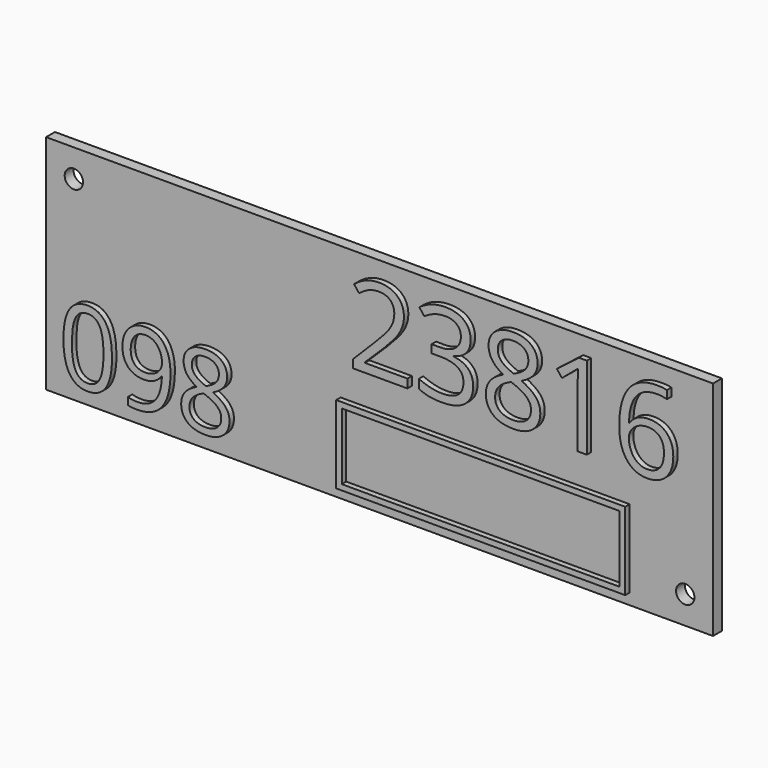
from build123d import *

# Parameters (mm, degrees)
F0_W         = 120
F0_H         = 40
F1_DEPTH     = 2
F3_D         = 3.3
F4_TEXT_SIZE = 20.871833895
F5_DEPTH     = 1
F6_TEXT_SIZE = 18.5155049272
F7_DEPTH     = 1
F8_W         = 52
F8_H         = 14
F8_W_2       = 49.99999962
F8_H_2       = 11.99999962
F9_DEPTH     = 1


# Not quite as in the source:
# - Text() gives the source's letters only with a copy of the font that has no kerning and outlines rounded to 1/6400 em; it was checked with that copy


with BuildPart() as f1:
    # F0 (on Front) → F1 (new body)
    with BuildSketch(Plane.XZ):
        Rectangle(F0_W, F0_H)
    extrude(amount=F1_DEPTH)

    # F3 (through all)
    with Locations(Plane.XZ.offset(2)):
        with Locations((-55, 15), (55, -15)):
            Hole(F3_D / 2)

    # F4 (on face) → F5 (join)
    with BuildSketch(Plane.XZ.offset(2)):
        with Locations((-5, 2)):
            Text('23816', F4_TEXT_SIZE, font='Open Sans', text_align=(TextAlign.LEFT, TextAlign.BOTTOM))
    extrude(amount=F5_DEPTH)

    # F6 (on face) → F7 (join)
    with BuildSketch(Plane.XZ.offset(2)):
        with Locations((-57, -17)):
            Text('098', F6_TEXT_SIZE, font='Open Sans', text_align=(TextAlign.LEFT, TextAlign.BOTTOM))
    extrude(amount=F7_DEPTH)

    # F8 (on face) → F9 (join)
    with BuildSketch(Plane.XZ.offset(2)):
        with Locations((19, -11)):
            Rectangle(F8_W, F8_H)
        with Locations((19, -11)):
            Rectangle(F8_W_2, F8_H_2, mode=Mode.SUBTRACT)
    extrude(amount=F9_DEPTH)


solid = f1.part
